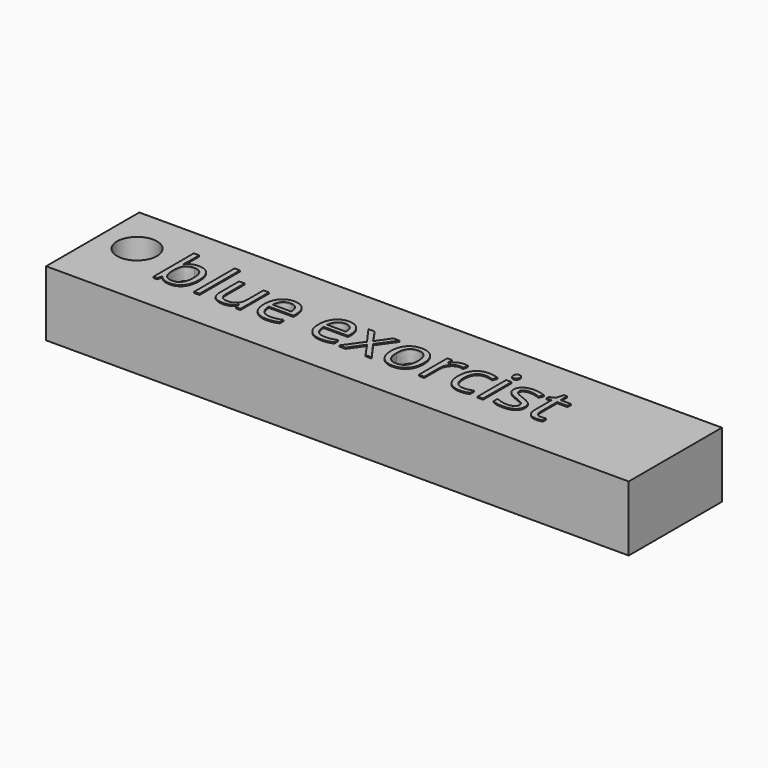
from build123d import *

# Parameters (mm, degrees)
F1_W         = 127
F1_H         = 25.4
F1_R         = 4.3560955088
F2_DEPTH     = 11.684
F3_W         = 127
F3_H         = 25.4
F3_W_2       = 1.1762167899
F3_H_2       = 7.7621242882
F3_R         = 4.3560955088
F3_H_3       = 11.0210833324
F3_TEXT_SIZE = 14.504407429
F4_DEPTH     = 2.54
F5_DEPTH     = 2.794


# Not quite as in the source:
# - Text() gives the source's letters only with a copy of the font that has no kerning and outlines rounded to 1/6400 em; it was checked with that copy


with BuildPart() as f2:
    # F1 (on face) → F2 (new body)
    with BuildSketch(Plane.XY):
        with Locations((29.9934654772, 32.9029177505)):
            Rectangle(F1_W, F1_H)
        with Locations((-25.4533998668, 34.9230393767)):
            Circle(F1_R, mode=Mode.SUBTRACT)
    extrude(amount=F2_DEPTH)

    # F3 (on face) → F4 (join)
    with BuildSketch(Plane.XY.offset(11.684)):
        with Locations((29.9934654772, 32.9029177505)):
            Rectangle(F3_W, F3_H)
        with BuildLine():
            Line((-4.0644988282, 35.9945683659), (-2.8746841563, 35.9945683659))
            Line((-2.8746841563, 35.9945683659), (-2.8746841563, 30.9588194117))
            add(Edge.make_bspline(
                [(-2.8746841563, 30.9588194117), (-2.8746841563, 30.0092339878), (-2.4429514039, 29.5423733737)],
                knots=[0, 0, 0, 1, 1, 1], degree=2))
            add(Edge.make_bspline(
                [(-2.4429514039, 29.5423733737), (-2.0112186515, 29.0755127595), (-1.0910953052, 29.0755127595)],
                knots=[0, 0, 0, 1, 1, 1], degree=2))
            add(Edge.make_bspline(
                [(-1.0910953052, 29.0755127595), (0.1281814443, 29.0755127595), (0.6902272321, 29.740675819)],
                knots=[0, 0, 0, 1, 1, 1], degree=2))
            add(Edge.make_bspline(
                [(0.6902272321, 29.740675819), (1.25227302, 30.4058388784), (1.25227302, 31.9152037765)],
                knots=[0, 0, 0, 1, 1, 1], degree=2))
            Line((1.25227302, 31.9152037765), (1.25227302, 35.9945683659))
            Line((1.25227302, 35.9945683659), (2.42848981, 35.9945683659))
            Line((2.42848981, 35.9945683659), (2.42848981, 28.2324440777))
            Line((2.42848981, 28.2324440777), (1.4585075632, 28.2324440777))
            Line((1.4585075632, 28.2324440777), (1.2885340386, 29.272682048))
            Line((1.2885340386, 29.272682048), (1.2250772561, 29.272682048))
            add(Edge.make_bspline(
                [(1.2250772561, 29.272682048), (0.864733384, 28.6993046919), (0.223366618, 28.3944855045)],
                knots=[0, 0, 0, 1, 1, 1], degree=2))
            add(Edge.make_bspline(
                [(0.223366618, 28.3944855045), (-0.418000148, 28.0896663171), (-1.2406720068, 28.0896663171)],
                knots=[0, 0, 0, 1, 1, 1], degree=2))
            add(Edge.make_bspline(
                [(-1.2406720068, 28.0896663171), (-2.6571180448, 28.0896663171), (-3.3608084365, 28.7627614744)],
                knots=[0, 0, 0, 1, 1, 1], degree=2))
            add(Edge.make_bspline(
                [(-3.3608084365, 28.7627614744), (-4.0644988282, 29.4358566316), (-4.0644988282, 30.9157594521)],
                knots=[0, 0, 0, 1, 1, 1], degree=2))
            Line((-4.0644988282, 30.9157594521), (-4.0644988282, 35.9945683659))
        make_face(mode=Mode.SUBTRACT)
        with BuildLine():
            add(Edge.make_bspline(
                [(9.5424483912, 28.2075146275), (8.9872015443, 28.0896663171), (8.200790704, 28.0896663171)],
                knots=[0, 0, 0, 1, 1, 1], degree=2))
            add(Edge.make_bspline(
                [(8.200790704, 28.0896663171), (6.4806586355, 28.0896663171), (5.4846137815, 29.138969542)],
                knots=[0, 0, 0, 1, 1, 1], degree=2))
            add(Edge.make_bspline(
                [(5.4846137815, 29.138969542), (4.4885689276, 30.188272767), (4.4885689276, 32.0489162825)],
                knots=[0, 0, 0, 1, 1, 1], degree=2))
            add(Edge.make_bspline(
                [(4.4885689276, 32.0489162825), (4.4885689276, 33.9276903073), (5.4132249012, 35.0325182169)],
                knots=[0, 0, 0, 1, 1, 1], degree=2))
            add(Edge.make_bspline(
                [(5.4132249012, 35.0325182169), (6.3378808748, 36.1373461266), (7.8971046735, 36.1373461266)],
                knots=[0, 0, 0, 1, 1, 1], degree=2))
            add(Edge.make_bspline(
                [(7.8971046735, 36.1373461266), (9.3543443573, 36.1373461266), (10.2042119801, 35.1775622912)],
                knots=[0, 0, 0, 1, 1, 1], degree=2))
            add(Edge.make_bspline(
                [(10.2042119801, 35.1775622912), (11.0540796029, 34.2177784559), (11.0540796029, 32.6449567753)],
                knots=[0, 0, 0, 1, 1, 1], degree=2))
            Line((11.0540796029, 32.6449567753), (11.0540796029, 31.9016058945))
            Line((11.0540796029, 31.9016058945), (5.7078456771, 31.9016058945))
            add(Edge.make_bspline(
                [(5.7078456771, 31.9016058945), (5.7441066957, 30.5350187571), (6.3990713437, 29.8267957381)],
                knots=[0, 0, 0, 1, 1, 1], degree=2))
            add(Edge.make_bspline(
                [(6.3990713437, 29.8267957381), (7.0540359916, 29.1185727191), (8.2438506636, 29.1185727191)],
                knots=[0, 0, 0, 1, 1, 1], degree=2))
            add(Edge.make_bspline(
                [(8.2438506636, 29.1185727191), (9.497122118, 29.1185727191), (10.7209314948, 29.6420911747)],
                knots=[0, 0, 0, 1, 1, 1], degree=2))
            Line((10.7209314948, 29.6420911747), (10.7209314948, 28.5927879498))
            add(Edge.make_bspline(
                [(10.7209314948, 28.5927879498), (10.0976952381, 28.3253629378), (9.5424483912, 28.2075146275)],
                knots=[0, 0, 0, 1, 1, 1], degree=2))
        make_face(mode=Mode.SUBTRACT)
        with BuildLine():
            add(Edge.make_bspline(
                [(21.449660365, 28.2075146275), (20.8944135181, 28.0896663171), (20.1080026778, 28.0896663171)],
                knots=[0, 0, 0, 1, 1, 1], degree=2))
            add(Edge.make_bspline(
                [(20.1080026778, 28.0896663171), (18.3878706092, 28.0896663171), (17.3918257553, 29.138969542)],
                knots=[0, 0, 0, 1, 1, 1], degree=2))
            add(Edge.make_bspline(
                [(17.3918257553, 29.138969542), (16.3957809014, 30.188272767), (16.3957809014, 32.0489162825)],
                knots=[0, 0, 0, 1, 1, 1], degree=2))
            add(Edge.make_bspline(
                [(16.3957809014, 32.0489162825), (16.3957809014, 33.9276903073), (17.320436875, 35.0325182169)],
                knots=[0, 0, 0, 1, 1, 1], degree=2))
            add(Edge.make_bspline(
                [(17.320436875, 35.0325182169), (18.2450928486, 36.1373461266), (19.8043166472, 36.1373461266)],
                knots=[0, 0, 0, 1, 1, 1], degree=2))
            add(Edge.make_bspline(
                [(19.8043166472, 36.1373461266), (21.2615563311, 36.1373461266), (22.1114239539, 35.1775622912)],
                knots=[0, 0, 0, 1, 1, 1], degree=2))
            add(Edge.make_bspline(
                [(22.1114239539, 35.1775622912), (22.9612915767, 34.2177784559), (22.9612915767, 32.6449567753)],
                knots=[0, 0, 0, 1, 1, 1], degree=2))
            Line((22.9612915767, 32.6449567753), (22.9612915767, 31.9016058945))
            Line((22.9612915767, 31.9016058945), (17.6150576509, 31.9016058945))
            add(Edge.make_bspline(
                [(17.6150576509, 31.9016058945), (17.6513186695, 30.5350187571), (18.3062833174, 29.8267957381)],
                knots=[0, 0, 0, 1, 1, 1], degree=2))
            add(Edge.make_bspline(
                [(18.3062833174, 29.8267957381), (18.9612479654, 29.1185727191), (20.1510626373, 29.1185727191)],
                knots=[0, 0, 0, 1, 1, 1], degree=2))
            add(Edge.make_bspline(
                [(20.1510626373, 29.1185727191), (21.4043340917, 29.1185727191), (22.6281434686, 29.6420911747)],
                knots=[0, 0, 0, 1, 1, 1], degree=2))
            Line((22.6281434686, 29.6420911747), (22.6281434686, 28.5927879498))
            add(Edge.make_bspline(
                [(22.6281434686, 28.5927879498), (22.0049072118, 28.3253629378), (21.449660365, 28.2075146275)],
                knots=[0, 0, 0, 1, 1, 1], degree=2))
        make_face(mode=Mode.SUBTRACT)
        Polygon((23.9969969197, 28.2324440777), (26.8366879366, 32.2052919251), (24.1375083666, 35.9945683659), (25.4768997402, 35.9945683659), (27.5233809759, 33.021164843), (29.5630632706, 35.9945683659), (30.8888567621, 35.9945683659), (28.1896771921, 32.2052919251), (31.0293682091, 28.2324440777), (29.6990420902, 28.2324440777), (27.5233809759, 31.3780874389), (25.3273230386, 28.2324440777), align=None, mode=Mode.SUBTRACT)
        with BuildLine():
            add(Edge.make_bspline(
                [(38.3053682171, 35.0529150399), (39.2651520524, 33.9684839532), (39.2651520524, 32.1214383196)],
                knots=[0, 0, 0, 1, 1, 1], degree=2))
            add(Edge.make_bspline(
                [(39.2651520524, 32.1214383196), (39.2651520524, 30.2222674719), (38.3099008444, 29.1559668945)],
                knots=[0, 0, 0, 1, 1, 1], degree=2))
            add(Edge.make_bspline(
                [(38.3099008444, 29.1559668945), (37.3546496364, 28.0896663171), (35.6685122727, 28.0896663171)],
                knots=[0, 0, 0, 1, 1, 1], degree=2))
            add(Edge.make_bspline(
                [(35.6685122727, 28.0896663171), (34.6260079888, 28.0896663171), (33.8192003255, 28.5791900678)],
                knots=[0, 0, 0, 1, 1, 1], degree=2))
            add(Edge.make_bspline(
                [(33.8192003255, 28.5791900678), (33.0123926623, 29.0687138186), (32.5727278121, 29.9820382239)],
                knots=[0, 0, 0, 1, 1, 1], degree=2))
            add(Edge.make_bspline(
                [(32.5727278121, 29.9820382239), (32.1330629619, 30.8953626292), (32.1330629619, 32.1214383196)],
                knots=[0, 0, 0, 1, 1, 1], degree=2))
            add(Edge.make_bspline(
                [(32.1330629619, 32.1214383196), (32.1330629619, 34.0183428537), (33.0826483858, 35.0778444901)],
                knots=[0, 0, 0, 1, 1, 1], degree=2))
            add(Edge.make_bspline(
                [(33.0826483858, 35.0778444901), (34.0322338096, 36.1373461266), (35.7183711733, 36.1373461266)],
                knots=[0, 0, 0, 1, 1, 1], degree=2))
            add(Edge.make_bspline(
                [(35.7183711733, 36.1373461266), (37.3455843817, 36.1373461266), (38.3053682171, 35.0529150399)],
                knots=[0, 0, 0, 1, 1, 1], degree=2))
        make_face(mode=Mode.SUBTRACT)
        with BuildLine():
            add(Edge.make_bspline(
                [(43.530354362, 35.7260101971), (44.1399927367, 36.1373461266), (44.8697457355, 36.1373461266)],
                knots=[0, 0, 0, 1, 1, 1], degree=2))
            add(Edge.make_bspline(
                [(44.8697457355, 36.1373461266), (45.3864652502, 36.1373461266), (45.7966680228, 36.0512262074)],
                knots=[0, 0, 0, 1, 1, 1], degree=2))
            Line((45.7966680228, 36.0512262074), (45.6334934392, 34.9611293366))
            add(Edge.make_bspline(
                [(45.6334934392, 34.9611293366), (45.1530349431, 35.0676460787), (44.7836258164, 35.0676460787)],
                knots=[0, 0, 0, 1, 1, 1], degree=2))
            add(Edge.make_bspline(
                [(44.7836258164, 35.0676460787), (43.8408393335, 35.0676460787), (43.1722768036, 34.3027652181)],
                knots=[0, 0, 0, 1, 1, 1], degree=2))
            add(Edge.make_bspline(
                [(43.1722768036, 34.3027652181), (42.5037142737, 33.5378843576), (42.5037142737, 32.3979285863)],
                knots=[0, 0, 0, 1, 1, 1], degree=2))
            Line((42.5037142737, 32.3979285863), (42.5037142737, 28.2324440777))
            Line((42.5037142737, 28.2324440777), (41.3274974837, 28.2324440777))
            Line((41.3274974837, 28.2324440777), (41.3274974837, 35.9945683659))
            Line((41.3274974837, 35.9945683659), (42.2974797305, 35.9945683659))
            Line((42.2974797305, 35.9945683659), (42.4334585502, 34.557725505))
            Line((42.4334585502, 34.557725505), (42.4901163917, 34.557725505))
            add(Edge.make_bspline(
                [(42.4901163917, 34.557725505), (42.9207159872, 35.3146742677), (43.530354362, 35.7260101971)],
                knots=[0, 0, 0, 1, 1, 1], degree=2))
        make_face(mode=Mode.SUBTRACT)
        with BuildLine():
            add(Edge.make_bspline(
                [(52.3123197975, 28.4953364624), (51.5349742119, 28.0896663171), (50.351958481, 28.0896663171)],
                knots=[0, 0, 0, 1, 1, 1], degree=2))
            add(Edge.make_bspline(
                [(50.351958481, 28.0896663171), (48.6658211173, 28.0896663171), (47.7411651437, 29.1276379737)],
                knots=[0, 0, 0, 1, 1, 1], degree=2))
            add(Edge.make_bspline(
                [(47.7411651437, 29.1276379737), (46.8165091701, 30.1656096304), (46.8165091701, 32.0647804781)],
                knots=[0, 0, 0, 1, 1, 1], degree=2))
            add(Edge.make_bspline(
                [(46.8165091701, 32.0647804781), (46.8165091701, 34.0115439127), (47.7558961825, 35.0744450196)],
                knots=[0, 0, 0, 1, 1, 1], degree=2))
            add(Edge.make_bspline(
                [(47.7558961825, 35.0744450196), (48.6952831949, 36.1373461266), (50.4290131454, 36.1373461266)],
                knots=[0, 0, 0, 1, 1, 1], degree=2))
            add(Edge.make_bspline(
                [(50.4290131454, 36.1373461266), (50.9887926196, 36.1373461266), (51.5485720939, 36.0160983457)],
                knots=[0, 0, 0, 1, 1, 1], degree=2))
            add(Edge.make_bspline(
                [(51.5485720939, 36.0160983457), (52.1083515681, 35.8948505648), (52.4256354806, 35.7316759813)],
                knots=[0, 0, 0, 1, 1, 1], degree=2))
            Line((52.4256354806, 35.7316759813), (52.0652916085, 34.7344979705))
            add(Edge.make_bspline(
                [(52.0652916085, 34.7344979705), (51.6754856589, 34.8908736131), (51.2154239857, 34.9928577279)],
                knots=[0, 0, 0, 1, 1, 1], degree=2))
            add(Edge.make_bspline(
                [(51.2154239857, 34.9928577279), (50.7553623126, 35.0948418426), (50.4018173815, 35.0948418426)],
                knots=[0, 0, 0, 1, 1, 1], degree=2))
            add(Edge.make_bspline(
                [(50.4018173815, 35.0948418426), (48.0357859196, 35.0948418426), (48.0357859196, 32.0783783601)],
                knots=[0, 0, 0, 1, 1, 1], degree=2))
            add(Edge.make_bspline(
                [(48.0357859196, 32.0783783601), (48.0357859196, 30.6483344401), (48.6125627463, 29.8834535796)],
                knots=[0, 0, 0, 1, 1, 1], degree=2))
            add(Edge.make_bspline(
                [(48.6125627463, 29.8834535796), (49.189339573, 29.1185727191), (50.3224964034, 29.1185727191)],
                knots=[0, 0, 0, 1, 1, 1], degree=2))
            add(Edge.make_bspline(
                [(50.3224964034, 29.1185727191), (51.2924786502, 29.1185727191), (52.3123197975, 29.5355744327)],
                knots=[0, 0, 0, 1, 1, 1], degree=2))
            Line((52.3123197975, 29.5355744327), (52.3123197975, 28.4953364624))
        make_face(mode=Mode.SUBTRACT)
        with Locations((54.7429411987, 32.1135062218)):
            Rectangle(F3_W_2, F3_H_2, mode=Mode.SUBTRACT)
        with BuildLine():
            add(Edge.make_bspline(
                [(62.3452903738, 31.6319145689), (62.8302814973, 31.1219939952), (62.8302814973, 30.3491810369)],
                knots=[0, 0, 0, 1, 1, 1], degree=2))
            add(Edge.make_bspline(
                [(62.8302814973, 30.3491810369), (62.8302814973, 29.265883107), (62.023473834, 28.6777747121)],
                knots=[0, 0, 0, 1, 1, 1], degree=2))
            add(Edge.make_bspline(
                [(62.023473834, 28.6777747121), (61.2166661708, 28.0896663171), (59.7571601732, 28.0896663171)],
                knots=[0, 0, 0, 1, 1, 1], degree=2))
            add(Edge.make_bspline(
                [(59.7571601732, 28.0896663171), (58.2138005702, 28.0896663171), (57.3503350655, 28.5791900678)],
                knots=[0, 0, 0, 1, 1, 1], degree=2))
            Line((57.3503350655, 28.5791900678), (57.3503350655, 29.6692869387))
            add(Edge.make_bspline(
                [(57.3503350655, 29.6692869387), (57.9101145397, 29.3859977311), (58.5503481489, 29.2239563043)],
                knots=[0, 0, 0, 1, 1, 1], degree=2))
            add(Edge.make_bspline(
                [(58.5503481489, 29.2239563043), (59.190581758, 29.0619148776), (59.7866222508, 29.0619148776)],
                knots=[0, 0, 0, 1, 1, 1], degree=2))
            add(Edge.make_bspline(
                [(59.7866222508, 29.0619148776), (60.7067455971, 29.0619148776), (61.201935132, 29.3554024966)],
                knots=[0, 0, 0, 1, 1, 1], degree=2))
            add(Edge.make_bspline(
                [(61.201935132, 29.3554024966), (61.6971246669, 29.6488901157), (61.6971246669, 30.2517295495)],
                knots=[0, 0, 0, 1, 1, 1], degree=2))
            add(Edge.make_bspline(
                [(61.6971246669, 30.2517295495), (61.6971246669, 30.7049922816), (61.3050524035, 31.0268088215)],
                knots=[0, 0, 0, 1, 1, 1], degree=2))
            add(Edge.make_bspline(
                [(61.3050524035, 31.0268088215), (60.9129801402, 31.3486253613), (59.7707580552, 31.7882902115)],
                knots=[0, 0, 0, 1, 1, 1], degree=2))
            add(Edge.make_bspline(
                [(59.7707580552, 31.7882902115), (58.6874601253, 32.1916940431), (58.2307979227, 32.49311376)],
                knots=[0, 0, 0, 1, 1, 1], degree=2))
            add(Edge.make_bspline(
                [(58.2307979227, 32.49311376), (57.77413572, 32.7945334769), (57.5509038244, 33.1764073287)],
                knots=[0, 0, 0, 1, 1, 1], degree=2))
            add(Edge.make_bspline(
                [(57.5509038244, 33.1764073287), (57.3276719289, 33.5582811806), (57.3276719289, 34.0885985772)],
                knots=[0, 0, 0, 1, 1, 1], degree=2))
            add(Edge.make_bspline(
                [(57.3276719289, 34.0885985772), (57.3276719289, 35.0381840011), (58.1004848872, 35.5877650638)],
                knots=[0, 0, 0, 1, 1, 1], degree=2))
            add(Edge.make_bspline(
                [(58.1004848872, 35.5877650638), (58.8732978455, 36.1373461266), (60.2172218464, 36.1373461266)],
                knots=[0, 0, 0, 1, 1, 1], degree=2))
            add(Edge.make_bspline(
                [(60.2172218464, 36.1373461266), (61.4704933008, 36.1373461266), (62.6693732273, 35.6274255529)],
                knots=[0, 0, 0, 1, 1, 1], degree=2))
            Line((62.6693732273, 35.6274255529), (62.2501052001, 34.671041188))
            add(Edge.make_bspline(
                [(62.2501052001, 34.671041188), (61.0829536648, 35.1514996841), (60.1333682409, 35.1514996841)],
                knots=[0, 0, 0, 1, 1, 1], degree=2))
            add(Edge.make_bspline(
                [(60.1333682409, 35.1514996841), (59.2970985001, 35.1514996841), (58.8721646887, 34.8897404563)],
                knots=[0, 0, 0, 1, 1, 1], degree=2))
            add(Edge.make_bspline(
                [(58.8721646887, 34.8897404563), (58.4472308773, 34.6279812285), (58.4472308773, 34.1679195553)],
                knots=[0, 0, 0, 1, 1, 1], degree=2))
            add(Edge.make_bspline(
                [(58.4472308773, 34.1679195553), (58.4472308773, 33.8551682701), (58.6070059904, 33.6364690019)],
                knots=[0, 0, 0, 1, 1, 1], degree=2))
            add(Edge.make_bspline(
                [(58.6070059904, 33.6364690019), (58.7667811035, 33.4177697336), (59.1203260345, 33.2194672883)],
                knots=[0, 0, 0, 1, 1, 1], degree=2))
            add(Edge.make_bspline(
                [(59.1203260345, 33.2194672883), (59.4738709656, 33.021164843), (60.480114231, 32.6449567753)],
                knots=[0, 0, 0, 1, 1, 1], degree=2))
            add(Edge.make_bspline(
                [(60.480114231, 32.6449567753), (61.8602992504, 32.1418351426), (62.3452903738, 31.6319145689)],
                knots=[0, 0, 0, 1, 1, 1], degree=2))
        make_face(mode=Mode.SUBTRACT)
        with Locations((-25.4533998668, 34.9230393767)):
            Circle(F3_R, mode=Mode.SUBTRACT)
        with BuildLine():
            add(Edge.make_bspline(
                [(-15.3620724272, 34.9611293366), (-14.541666882, 36.1214819309), (-12.9257852419, 36.1214819309)],
                knots=[0, 0, 0, 1, 1, 1], degree=2))
            add(Edge.make_bspline(
                [(-12.9257852419, 36.1214819309), (-11.3960235208, 36.1214819309), (-10.5495553685, 35.0767113333)],
                knots=[0, 0, 0, 1, 1, 1], degree=2))
            add(Edge.make_bspline(
                [(-10.5495553685, 35.0767113333), (-9.7030872162, 34.0319407357), (-9.7030872162, 32.1214383196)],
                knots=[0, 0, 0, 1, 1, 1], degree=2))
            add(Edge.make_bspline(
                [(-9.7030872162, 32.1214383196), (-9.7030872162, 30.2086695899), (-10.5563543095, 29.1491679535)],
                knots=[0, 0, 0, 1, 1, 1], degree=2))
            add(Edge.make_bspline(
                [(-10.5563543095, 29.1491679535), (-11.4096214028, 28.0896663171), (-12.9257852419, 28.0896663171)],
                knots=[0, 0, 0, 1, 1, 1], degree=2))
            add(Edge.make_bspline(
                [(-12.9257852419, 28.0896663171), (-13.6850003182, 28.0896663171), (-14.3116360454, 28.3695560542)],
                knots=[0, 0, 0, 1, 1, 1], degree=2))
            add(Edge.make_bspline(
                [(-14.3116360454, 28.3695560542), (-14.9382717726, 28.6494457913), (-15.3620724272, 29.2318884021)],
                knots=[0, 0, 0, 1, 1, 1], degree=2))
            Line((-15.3620724272, 29.2318884021), (-15.4481923463, 29.2318884021))
            Line((-15.4481923463, 29.2318884021), (-15.6952205353, 28.2324440777))
            Line((-15.6952205353, 28.2324440777), (-16.5382892171, 28.2324440777))
            Line((-16.5382892171, 28.2324440777), (-16.5382892171, 39.2535274101))
            Line((-16.5382892171, 39.2535274101), (-15.3620724272, 39.2535274101))
            Line((-15.3620724272, 39.2535274101), (-15.3620724272, 36.5747446631))
            add(Edge.make_bspline(
                [(-15.3620724272, 36.5747446631), (-15.3620724272, 35.6750181398), (-15.4187302687, 34.9611293366)],
                knots=[0, 0, 0, 1, 1, 1], degree=2))
            Line((-15.4187302687, 34.9611293366), (-15.3620724272, 34.9611293366))
        make_face(mode=Mode.SUBTRACT)
        with Locations((-7.0616986446, 33.7429857439)):
            Rectangle(F3_W_2, F3_H_3, mode=Mode.SUBTRACT)
        with BuildLine():
            add(Edge.make_bspline(
                [(54.253417448, 37.5061995777), (54.0551150027, 37.7011025525), (54.0551150027, 38.0977074431)],
                knots=[0, 0, 0, 1, 1, 1], degree=2))
            add(Edge.make_bspline(
                [(54.0551150027, 38.0977074431), (54.0551150027, 38.5011112748), (54.253417448, 38.6892153086)],
                knots=[0, 0, 0, 1, 1, 1], degree=2))
            add(Edge.make_bspline(
                [(54.253417448, 38.6892153086), (54.4517198933, 38.8773193424), (54.7508732965, 38.8773193424)],
                knots=[0, 0, 0, 1, 1, 1], degree=2))
            add(Edge.make_bspline(
                [(54.7508732965, 38.8773193424), (55.0341625041, 38.8773193424), (55.2392638904, 38.6858158381)],
                knots=[0, 0, 0, 1, 1, 1], degree=2))
            add(Edge.make_bspline(
                [(55.2392638904, 38.6858158381), (55.4443652767, 38.4943123338), (55.4443652767, 38.0977074431)],
                knots=[0, 0, 0, 1, 1, 1], degree=2))
            add(Edge.make_bspline(
                [(55.4443652767, 38.0977074431), (55.4443652767, 37.7011025525), (55.2392638904, 37.5061995777)],
                knots=[0, 0, 0, 1, 1, 1], degree=2))
            add(Edge.make_bspline(
                [(55.2392638904, 37.5061995777), (55.0341625041, 37.3112966028), (54.7508732965, 37.3112966028)],
                knots=[0, 0, 0, 1, 1, 1], degree=2))
            add(Edge.make_bspline(
                [(54.7508732965, 37.3112966028), (54.4517198933, 37.3112966028), (54.253417448, 37.5061995777)],
                knots=[0, 0, 0, 1, 1, 1], degree=2))
        make_face(mode=Mode.SUBTRACT)
        with BuildLine():
            add(Edge.make_bspline(
                [(66.3362687305, 29.4369897884), (66.6694168386, 29.0619148776), (67.2495931358, 29.0619148776)],
                knots=[0, 0, 0, 1, 1, 1], degree=2))
            add(Edge.make_bspline(
                [(67.2495931358, 29.0619148776), (67.562344421, 29.0619148776), (67.8524325696, 29.1072411508)],
                knots=[0, 0, 0, 1, 1, 1], degree=2))
            add(Edge.make_bspline(
                [(67.8524325696, 29.1072411508), (68.1425207181, 29.152567424), (68.3124942427, 29.2024263245)],
                knots=[0, 0, 0, 1, 1, 1], degree=2))
            Line((68.3124942427, 29.2024263245), (68.3124942427, 28.3026998012))
            add(Edge.make_bspline(
                [(68.3124942427, 28.3026998012), (68.1221238952, 28.2120472548), (67.7504484548, 28.1508567859)],
                knots=[0, 0, 0, 1, 1, 1], degree=2))
            add(Edge.make_bspline(
                [(67.7504484548, 28.1508567859), (67.3787730144, 28.0896663171), (67.0796196112, 28.0896663171)],
                knots=[0, 0, 0, 1, 1, 1], degree=2))
            add(Edge.make_bspline(
                [(67.0796196112, 28.0896663171), (64.8291701461, 28.0896663171), (64.8291701461, 30.4624967199)],
                knots=[0, 0, 0, 1, 1, 1], degree=2))
            Line((64.8291701461, 30.4624967199), (64.8291701461, 35.0812439606))
            Line((64.8291701461, 35.0812439606), (63.7164101386, 35.0812439606))
            Line((63.7164101386, 35.0812439606), (63.7164101386, 35.6478223758))
            Line((63.7164101386, 35.6478223758), (64.8291701461, 36.1373461266))
            Line((64.8291701461, 36.1373461266), (65.3232265241, 37.7940214126))
            Line((65.3232265241, 37.7940214126), (66.0031206224, 37.7940214126))
            Line((66.0031206224, 37.7940214126), (66.0031206224, 35.9945683659))
            Line((66.0031206224, 35.9945683659), (68.2558364012, 35.9945683659))
            Line((68.2558364012, 35.9945683659), (68.2558364012, 35.0812439606))
            Line((68.2558364012, 35.0812439606), (66.0031206224, 35.0812439606))
            Line((66.0031206224, 35.0812439606), (66.0031206224, 30.5123556205))
            add(Edge.make_bspline(
                [(66.0031206224, 30.5123556205), (66.0031206224, 29.8120646993), (66.3362687305, 29.4369897884)],
                knots=[0, 0, 0, 1, 1, 1], degree=2))
        make_face(mode=Mode.SUBTRACT)
        with Locations((-17.7847617306, 28.2324440777)):
            Text('blue exorcist', F3_TEXT_SIZE, font='Open Sans', text_align=(TextAlign.LEFT, TextAlign.BOTTOM))
    extrude(amount=F4_DEPTH)

    # F3 (on face) → F5 (join)
    with BuildSketch(Plane.XY.offset(11.684)):
        with Locations((-17.7847617306, 28.2324440777)):
            Text('blue exorcist', F3_TEXT_SIZE, font='Open Sans', text_align=(TextAlign.LEFT, TextAlign.BOTTOM))
    extrude(amount=F5_DEPTH)


solid = f2.part
